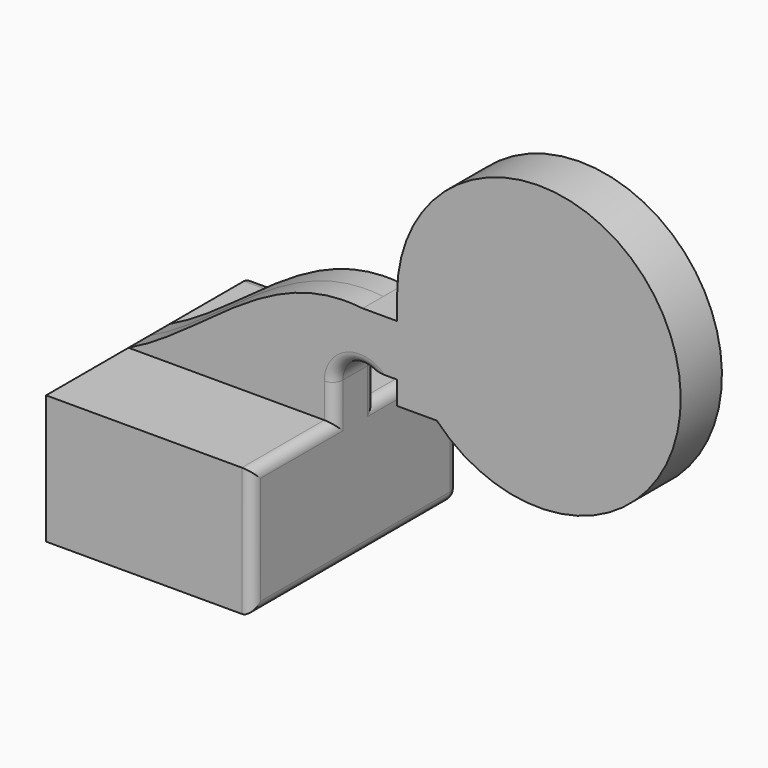
from build123d import *

# Parameters (mm, degrees)
F1_DEPTH     = 63.5
F2_DEPTH     = 12.7
F2_FACE_W    = 69.919578209
F2_FACE_H    = 25.4
F4_T1_DEPTH  = 134.62
F4_T3_DEPTH  = 53.34
F4_T5_DEPTH  = 45.72
F4_T7_DEPTH  = 16.9064607487
F4_T9_DEPTH  = 63.5
F4_T11_DEPTH = 88.9
F4_T13_DEPTH = 109.22
F4_S17_W     = 5.08
F4_S17_H     = 5.08
F4_T18_DEPTH = 5.08
F4_S23_W     = 5.08
F4_S23_H     = 5.08
F4_T24_DEPTH = 5.08
F4_T28_ANGLE = 152.7793054157
F4_T30_ANGLE = 152.7793054157
F4_T35_DEPTH = 58.42
F4_T39_DEPTH = 29.6064607487
F4_T46_DEPTH = 76.2
F4_T50_DEPTH = 29.6064607487


# Not quite as in the source:
# - a fillet or chamfer that OpenCascade refuses, or shapes differently, is made with other operations: its cross-section is extruded or revolved along the edge and cut away or added


with BuildPart() as f1:
    # F0 (on Front) → F1 (new body, symmetric)
    with BuildSketch(Plane.XZ):
        Polygon((-50.8, 31.75), (-50.8, -31.75), (50.8, -31.75), (50.8, 31.75), (25.4, 31.75), align=None)
    extrude(amount=F1_DEPTH, both=True)

    # F0 (on Front) → F2 (join, symmetric)
    with BuildSketch(Plane.XZ):
        with BuildLine():
            add(Edge.make_bspline(
                [(-50.8, 31.75), (-12.3217052749, 49.9639766453), (18.113411963, 91.8597280979), (64.6348841752, 86.3919299359)],
                knots=[0, 0, 0, 0, 127.7143413704, 127.7143413704, 127.7143413704, 127.7143413704], degree=3))
            Line((-50.8, 31.75), (25.4, 31.75))
            Line((25.4, 31.75), (25.4, 48.6564607487))
            ThreePointArc((25.4, 48.6564607487), (36.9860122893, 75.8747531778), (64.6348841752, 86.3919299359))
        make_face()
        with BuildLine():
            Line((25.4, 31.75), (50.8, 31.75))
            Line((50.8, 31.75), (50.8, 48.6564607487))
            ThreePointArc((50.8, 48.6564607487), (54.7240260068, 57.691740436), (64.0053517954, 60.9919299359))
            Line((64.0053517954, 60.9919299359), (81.6413929723, 60.9919299359))
            Line((81.6413929723, 60.9919299359), (81.6413929723, 86.3919299359))
            Line((81.6413929723, 86.3919299359), (64.6348841752, 86.3919299359))
            ThreePointArc((64.6348841752, 86.3919299359), (36.9860122893, 75.8747531778), (25.4, 48.6564607487))
            Line((25.4, 48.6564607487), (25.4, 31.75))
        make_face()
        Polygon((81.6413929723, 98.0887729745), (81.6413929723, 86.3919299359), (81.6413929723, 60.9919299359), (81.6413929723, 49.5563661095), (151.5609711813, 49.5563661095), (151.5609711813, 98.0887729745), align=None)
    extrude(amount=F2_DEPTH, both=True)

    # F2_face (on face) → F3 (revolve)
    with BuildSketch(Plane(origin=(116.6011820768, 0, 98.0887729745), x_dir=(1, 0, 0), z_dir=(0, 0, 1))):
        Rectangle(F2_FACE_W, F2_FACE_H)
    revolve(axis=Axis((151.5609711813, 0, 98.0887729745), (0, -1, 0)))

    # F4: fillet of radius 5.08 on 13 edges, made by hand

    # F4_s2 → F4_t1 (cut)
    with BuildSketch(Plane.XZ.offset(-58.42)):
        with BuildLine():
            ThreePointArc((45.72, -31.75), (49.3121024484, -30.2621024484), (50.8, -26.67))
            Line((50.8, -26.67), (50.8, -31.75))
            Line((50.8, -31.75), (45.72, -31.75))
        make_face()
    extrude(amount=F4_T1_DEPTH, mode=Mode.SUBTRACT)

    # F4_s4 → F4_t3 (cut)
    with BuildSketch(Plane.XY.offset(-26.67)):
        with BuildLine():
            ThreePointArc((45.72, 63.5), (49.3121024484, 62.0121024484), (50.8, 58.42))
            Line((50.8, 58.42), (50.8, 63.5))
            Line((50.8, 63.5), (45.72, 63.5))
        make_face()
    extrude(amount=F4_T3_DEPTH, mode=Mode.SUBTRACT)

    # F4_s6 → F4_t5 (cut)
    with BuildSketch(Plane.XZ.offset(-58.42)):
        with BuildLine():
            ThreePointArc((45.72, 31.75), (49.3121024484, 30.2621024484), (50.8, 26.67))
            Line((50.8, 26.67), (50.8, 31.75))
            Line((50.8, 31.75), (45.72, 31.75))
        make_face()
    extrude(amount=F4_T5_DEPTH, mode=Mode.SUBTRACT)

    # F4_s8 → F4_t7 (cut)
    with BuildSketch(Plane.XY.offset(31.75)):
        with BuildLine():
            ThreePointArc((50.8, 7.62), (49.3121024484, 11.2121024484), (45.72, 12.7))
            Line((45.72, 12.7), (50.8, 12.7))
            Line((50.8, 12.7), (50.8, 7.62))
        make_face()
        with BuildLine():
            ThreePointArc((50.8, -7.62), (49.3121024484, -11.2121024484), (45.72, -12.7))
            Line((45.72, -12.7), (50.8, -12.7))
            Line((50.8, -12.7), (50.8, -7.62))
        make_face()
    extrude(amount=F4_T7_DEPTH, mode=Mode.SUBTRACT)

    # F4_s10 → F4_t9 (cut)
    with BuildSketch(Plane.XZ.offset(12.7)):
        with BuildLine():
            ThreePointArc((45.72, 31.75), (49.3121024484, 30.2621024484), (50.8, 26.67))
            Line((50.8, 26.67), (50.8, 31.75))
            Line((50.8, 31.75), (45.72, 31.75))
        make_face()
    extrude(amount=F4_T9_DEPTH, mode=Mode.SUBTRACT)

    # F4_s12 → F4_t11 (cut)
    with BuildSketch(Plane.XY.offset(-44.45)):
        with BuildLine():
            ThreePointArc((45.72, -63.5), (49.3121024484, -62.0121024484), (50.8, -58.42))
            Line((50.8, -58.42), (50.8, -63.5))
            Line((50.8, -63.5), (45.72, -63.5))
        make_face()
        with BuildLine():
            ThreePointArc((-50.8, 58.42), (-49.3121024484, 62.0121024484), (-45.72, 63.5))
            Line((-45.72, 63.5), (-50.8, 63.5))
            Line((-50.8, 63.5), (-50.8, 58.42))
        make_face()
    extrude(amount=F4_T11_DEPTH, mode=Mode.SUBTRACT)

    # F4_s14 → F4_t13 (cut)
    with BuildSketch(Plane.YZ.offset(-63.5)):
        with BuildLine():
            ThreePointArc((63.5, -26.67), (62.0121024484, -30.2621024484), (58.42, -31.75))
            Line((58.42, -31.75), (63.5, -31.75))
            Line((63.5, -31.75), (63.5, -26.67))
        make_face()
        with BuildLine():
            ThreePointArc((63.5, 26.67), (62.0121024484, 30.2621024484), (58.42, 31.75))
            Line((58.42, 31.75), (63.5, 31.75))
            Line((63.5, 31.75), (63.5, 26.67))
        make_face()
    extrude(amount=F4_T13_DEPTH, mode=Mode.SUBTRACT)


with BuildPart() as f4_tool16:
    # F4_s17 → F4_t18 (new body)
    with BuildSketch(Plane.YZ.offset(45.72)):
        with Locations((60.96, -29.21)):
            Rectangle(F4_S17_W, F4_S17_H)
    extrude(amount=F4_T18_DEPTH)

    # F4_s19 → F4_t20 (revolve, cut)
    with BuildSketch(Plane(origin=(45.72, 58.42, -26.67), x_dir=(0, -0.7071067812, 0.7071067812), z_dir=(0, 0.7071067812, 0.7071067812))):
        with BuildLine():
            ThreePointArc((0, -5.08), (5.08, 0), (0, 5.08))
            Line((0, 5.08), (0, -5.08))
        make_face()
    revolve(axis=Axis((45.72, 58.42, -26.67), (1, 0, 0)), mode=Mode.SUBTRACT)


with BuildPart() as f1_1:
    add(f1.part)

    # F4_t15: cut F4_tool16
    add(f4_tool16.part, mode=Mode.SUBTRACT)


with BuildPart() as f4_tool22:
    # F4_s23 → F4_t24 (new body)
    with BuildSketch(Plane.YZ.offset(45.72)):
        with Locations((60.96, 29.21)):
            Rectangle(F4_S23_W, F4_S23_H)
    extrude(amount=F4_T24_DEPTH)

    # F4_s25 → F4_t26 (revolve, cut)
    with BuildSketch(Plane(origin=(45.72, 58.42, 26.67), x_dir=(0, -0.7071067812, -0.7071067812), z_dir=(0, -0.7071067812, 0.7071067812))):
        with BuildLine():
            ThreePointArc((0, -5.08), (5.08, 0), (0, 5.08))
            Line((0, 5.08), (0, -5.08))
        make_face()
    revolve(axis=Axis((45.72, 58.42, 26.67), (1, 0, 0)), mode=Mode.SUBTRACT)


with BuildPart() as f1_2:
    add(f1_1.part)

    # F4_t21: cut F4_tool22
    add(f4_tool22.part, mode=Mode.SUBTRACT)

    # F4_s27 → F4_t28 (revolve, cut)
    with BuildSketch(Plane.XY.offset(48.6564607487)):
        with BuildLine():
            ThreePointArc((45.72, -12.7), (49.3121024484, -11.2121024484), (50.8, -7.62))
            Line((50.8, -7.62), (50.8, -12.7))
            Line((50.8, -12.7), (45.72, -12.7))
        make_face()
    revolve(axis=Axis((63.1641202888, -12.7, 48.6564607487), (0, 1, 0)), revolution_arc=F4_T28_ANGLE, mode=Mode.SUBTRACT)

    # F4_s29 → F4_t30 (revolve, cut)
    with BuildSketch(Plane.XY.offset(48.6564607487)):
        with BuildLine():
            ThreePointArc((45.72, 12.7), (49.3121024484, 11.2121024484), (50.8, 7.62))
            Line((50.8, 7.62), (50.8, 12.7))
            Line((50.8, 12.7), (45.72, 12.7))
        make_face()
    revolve(axis=Axis((63.1641202888, 12.7, 48.6564607487), (0, 1, 0)), revolution_arc=F4_T30_ANGLE, mode=Mode.SUBTRACT)


with BuildPart() as f4_tool33:
    # F4_s34 → F4_t35 (new body)
    with BuildSketch(Plane.XZ):
        with BuildLine():
            ThreePointArc((45.72, 31.75), (49.3121024484, 30.2621024484), (50.8, 26.67))
            Line((50.8, 26.67), (50.8, 31.75))
            Line((50.8, 31.75), (45.72, 31.75))
        make_face()
    extrude(amount=-F4_T35_DEPTH)

    split(bisect_by=Plane.XZ.offset(-12.7), keep=Keep.TOP)


with BuildPart() as f4_tool37:
    # F4_s38 → F4_t39 (new body)
    with BuildSketch(Plane.XY.offset(19.05)):
        with BuildLine():
            ThreePointArc((50.8, 7.62), (49.3121024484, 11.2121024484), (45.72, 12.7))
            Line((45.72, 12.7), (50.8, 12.7))
            Line((50.8, 12.7), (50.8, 7.62))
        make_face()
    extrude(amount=F4_T39_DEPTH)

    split(bisect_by=Plane.XY.offset(31.75), keep=Keep.BOTTOM)


with BuildPart() as f4_tool33_1:
    add(f4_tool33.part)

    # F4_t41: intersect F4_tool37
    add(f4_tool37.part, mode=Mode.INTERSECT)


with BuildPart() as f1_3:
    add(f1_2.part)

    # F4_t31: cut F4_tool33
    add(f4_tool33_1.part, mode=Mode.SUBTRACT)


with BuildPart() as f4_tool44:
    # F4_s45 → F4_t46 (new body)
    with BuildSketch(Plane.XZ.offset(76.2)):
        with BuildLine():
            ThreePointArc((45.72, 31.75), (49.3121024484, 30.2621024484), (50.8, 26.67))
            Line((50.8, 26.67), (50.8, 31.75))
            Line((50.8, 31.75), (45.72, 31.75))
        make_face()
    extrude(amount=-F4_T46_DEPTH)

    split(bisect_by=Plane.XZ.offset(12.7), keep=Keep.BOTTOM)


with BuildPart() as f4_tool48:
    # F4_s49 → F4_t50 (new body)
    with BuildSketch(Plane.XY.offset(19.05)):
        with BuildLine():
            ThreePointArc((50.8, -7.62), (49.3121024484, -11.2121024484), (45.72, -12.7))
            Line((45.72, -12.7), (50.8, -12.7))
            Line((50.8, -12.7), (50.8, -7.62))
        make_face()
    extrude(amount=F4_T50_DEPTH)

    split(bisect_by=Plane.XY.offset(31.75), keep=Keep.BOTTOM)


with BuildPart() as f4_tool44_1:
    add(f4_tool44.part)

    # F4_t52: intersect F4_tool48
    add(f4_tool48.part, mode=Mode.INTERSECT)


with BuildPart() as f1_4:
    add(f1_3.part)

    # F4_t42: cut F4_tool44
    add(f4_tool44_1.part, mode=Mode.SUBTRACT)


solid = f1_4.part
